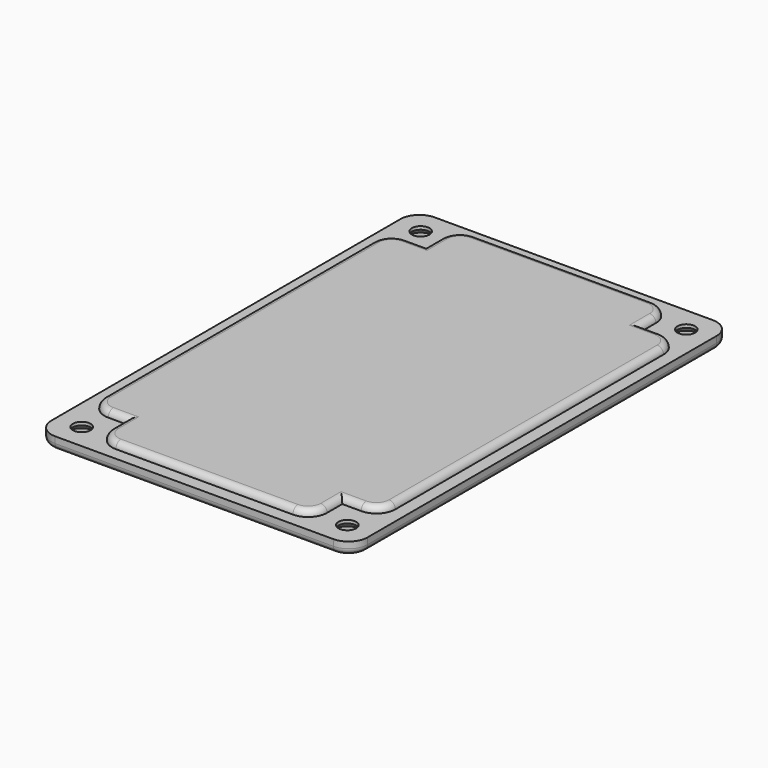
from build123d import *

# Parameters (mm, degrees)
F1_DEPTH      = 2
F2_R          = 1.4
F3_DEPTH      = 5
F5_DEPTH      = 1
F6_R          = 0.99999
F7_R          = 1
F8_R          = 2.25
F9_DEPTH      = 0.5
F10_S5_R      = 2.25
F10_T6_DEPTH  = 5
F10_S11_R     = 2.25
F10_T12_DEPTH = 5
F10_S17_R     = 2.25
F10_T18_DEPTH = 5
F10_S23_R     = 2.25
F10_T24_DEPTH = 5


# Not quite as in the source:
# - a fillet or chamfer that OpenCascade refuses, or shapes differently, is made with other operations: its cross-section is extruded or revolved along the edge and cut away or added
# - a fillet or chamfer is up to 0.001 mm smaller than in the source, because OpenCascade refuses the exact size


with BuildPart() as f1:
    # F0 (on Top) → F1 (new body)
    with BuildSketch(Plane.XY):
        with BuildLine():
            ThreePointArc((0, 3), (0.8786796564, 0.8786796564), (3, 0))
            Line((3, 0), (47, 0))
            ThreePointArc((47, 0), (49.1213203436, 0.8786796564), (50, 3))
            Line((50, 3), (50, 72))
            ThreePointArc((50, 72), (49.1213203436, 74.1213203436), (47, 75))
            Line((47, 75), (3, 75))
            ThreePointArc((3, 75), (0.8786796564, 74.1213203436), (0, 72))
            Line((0, 72), (0, 3))
        make_face()
    extrude(amount=F1_DEPTH)

    # F2 (on face) → F3 (cut)
    with BuildSketch(Plane.XY.offset(2)):
        with Locations((4, 71)):
            Circle(F2_R)
        with Locations((46, 71)):
            Circle(F2_R)
        with Locations((4, 4)):
            Circle(F2_R)
        with Locations((46, 4)):
            Circle(F2_R)
    extrude(amount=-F3_DEPTH, mode=Mode.SUBTRACT)

    # F4 (on face) → F5 (join)
    with BuildSketch(Plane.XY.offset(2)):
        with BuildLine():
            ThreePointArc((8, 5), (8.8786796564, 2.8786796564), (11, 2))
            Line((11, 2), (39, 2))
            ThreePointArc((39, 2), (41.1213203436, 2.8786796564), (42, 5))
            Line((42, 5), (42, 8))
            Line((42, 8), (45, 8))
            ThreePointArc((45, 8), (47.1213203436, 8.8786796564), (48, 11))
            Line((48, 11), (48, 64))
            ThreePointArc((48, 64), (47.1213203436, 66.1213203436), (45, 67))
            Line((45, 67), (42, 67))
            Line((42, 67), (42, 70))
            ThreePointArc((42, 70), (41.1213203436, 72.1213203436), (39, 73))
            Line((39, 73), (11, 73))
            ThreePointArc((11, 73), (8.8786796564, 72.1213203436), (8, 70))
            Line((8, 70), (8, 67))
            Line((8, 67), (5, 67))
            ThreePointArc((5, 67), (2.8786796564, 66.1213203436), (2, 64))
            Line((2, 64), (2, 11))
            ThreePointArc((2, 11), (2.8786796564, 8.8786796564), (5, 8))
            Line((5, 8), (8, 8))
            Line((8, 8), (8, 5))
        make_face()
    extrude(amount=F5_DEPTH)

    # F6 (radius 1 in the source; OpenCascade refuses exactly that, so slightly less here)
    f6_edges = [f1.edges().sort_by_distance(p)[0] for p in [
        (47.12132, 8.87868, 3),
        (43.5, 8, 3),
        (42, 6.5, 3),
        (41.12132, 2.87868, 3),
        (25, 2, 3),
        (8.87868, 2.87868, 3),
        (8, 6.5, 3),
        (6.5, 8, 3),
        (2.87868, 8.87868, 3),
        (2, 37.5, 3),
        (2.87868, 66.12132, 3),
        (6.5, 67, 3),
        (8, 68.5, 3),
        (8.87868, 72.12132, 3),
        (25, 73, 3),
        (41.12132, 72.12132, 3),
        (42, 68.5, 3),
        (43.5, 67, 3),
        (47.12132, 66.12132, 3),
        (48, 37.5, 3),
    ]]
    fillet(f6_edges, radius=F6_R)

    # F7
    f7_edges = [f1.edges().sort_by_distance(p)[0] for p in [
        (0, 37.5, 0),
    ]]
    fillet(f7_edges, radius=F7_R)

    # F8 (on face) → F9 (cut)
    with BuildSketch(Plane(origin=(0, 0, 0), x_dir=(1, 0, 0), z_dir=(0, 0, -1))):
        with Locations((4, -4)):
            Circle(F8_R)
        with Locations((46, -4)):
            Circle(F8_R)
        with Locations((46, -71)):
            Circle(F8_R)
        with Locations((4, -71)):
            Circle(F8_R)
    extrude(amount=-F9_DEPTH, mode=Mode.SUBTRACT)

    # F10: chamfer of 1 on 4 edges, made by hand


with BuildPart() as f10_tool2:
    # F10_s3 → F10_t4 (revolve)
    with BuildSketch(Plane.XZ.offset(-4)):
        Polygon((5.4, 1.5), (6.4, 0.5), (5.4, 0.5), align=None)
    revolve(axis=Axis((4, 4, 0.5), (0, 0, 1)))

    # F10_s5 → F10_t6 (intersect, symmetric)
    with BuildSketch(Plane.XY.offset(1)):
        with Locations((4, 4)):
            Circle(F10_S5_R)
    extrude(amount=F10_T6_DEPTH, both=True, mode=Mode.INTERSECT)


with BuildPart() as f1_1:
    add(f1.part)

    # F10_t1: cut F10_tool2
    add(f10_tool2.part, mode=Mode.SUBTRACT)


with BuildPart() as f10_tool8:
    # F10_s9 → F10_t10 (revolve)
    with BuildSketch(Plane.XZ.offset(-4)):
        Polygon((47.4, 1.5), (48.4, 0.5), (47.4, 0.5), align=None)
    revolve(axis=Axis((46, 4, 0.5), (0, 0, 1)))

    # F10_s11 → F10_t12 (intersect, symmetric)
    with BuildSketch(Plane.XY.offset(1)):
        with Locations((46, 4)):
            Circle(F10_S11_R)
    extrude(amount=F10_T12_DEPTH, both=True, mode=Mode.INTERSECT)


with BuildPart() as f1_2:
    add(f1_1.part)

    # F10_t7: cut F10_tool8
    add(f10_tool8.part, mode=Mode.SUBTRACT)


with BuildPart() as f10_tool14:
    # F10_s15 → F10_t16 (revolve)
    with BuildSketch(Plane.XZ.offset(-71)):
        Polygon((5.4, 1.5), (6.4, 0.5), (5.4, 0.5), align=None)
    revolve(axis=Axis((4, 71, 0.5), (0, 0, 1)))

    # F10_s17 → F10_t18 (intersect, symmetric)
    with BuildSketch(Plane.XY.offset(1)):
        with Locations((4, 71)):
            Circle(F10_S17_R)
    extrude(amount=F10_T18_DEPTH, both=True, mode=Mode.INTERSECT)


with BuildPart() as f1_3:
    add(f1_2.part)

    # F10_t13: cut F10_tool14
    add(f10_tool14.part, mode=Mode.SUBTRACT)


with BuildPart() as f10_tool20:
    # F10_s21 → F10_t22 (revolve)
    with BuildSketch(Plane.XZ.offset(-71)):
        Polygon((47.4, 1.5), (48.4, 0.5), (47.4, 0.5), align=None)
    revolve(axis=Axis((46, 71, 0.5), (0, 0, 1)))

    # F10_s23 → F10_t24 (intersect, symmetric)
    with BuildSketch(Plane.XY.offset(1)):
        with Locations((46, 71)):
            Circle(F10_S23_R)
    extrude(amount=F10_T24_DEPTH, both=True, mode=Mode.INTERSECT)


with BuildPart() as f1_4:
    add(f1_3.part)

    # F10_t19: cut F10_tool20
    add(f10_tool20.part, mode=Mode.SUBTRACT)


solid = f1_4.part
